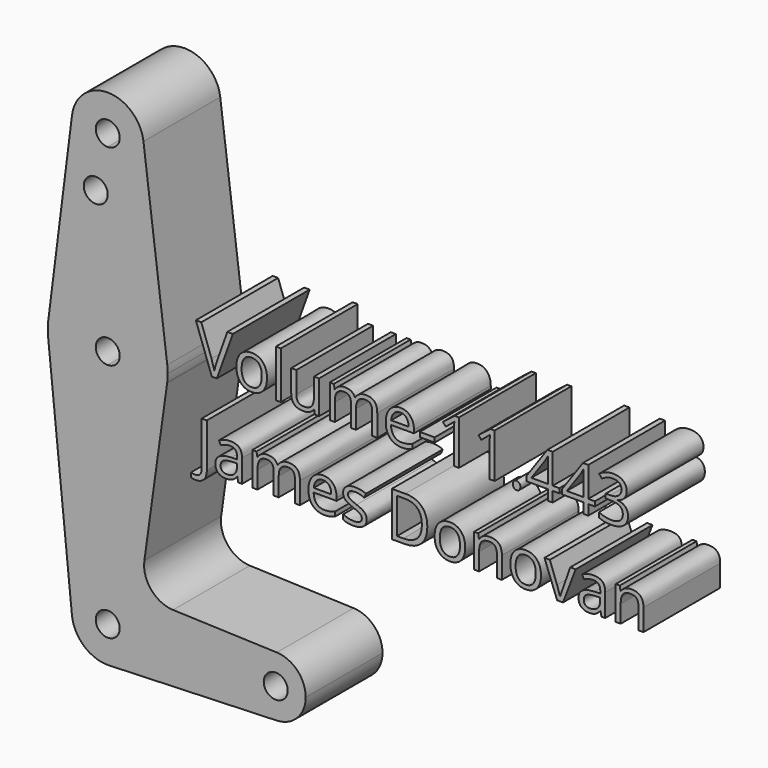
from build123d import *

# Parameters (mm, degrees)
F1_TEXT_SIZE = 16.465700335
F0_R         = 3.175
F2_DEPTH     = 25.4


# Not quite as in the source:
# - Text() gives the source's letters only with a copy of the font that has no kerning and outlines rounded to 1/6400 em; it was checked with that copy


with BuildPart() as f2:
    # F1 (on Front) + F0 (on Front) → F2 (new body)
    with BuildSketch(Plane.XZ):
        with Locations((-21.1360552348, 51.8487617373)):
            Text('Volume-11.443', F1_TEXT_SIZE, font='Open Sans', text_align=(TextAlign.LEFT, TextAlign.BOTTOM))
        with Locations((-21.1360552348, 29.4554092818)):
            Text('James Donovan', F1_TEXT_SIZE, font='Open Sans', text_align=(TextAlign.LEFT, TextAlign.BOTTOM))
    with BuildSketch(Plane.XZ):
        with BuildLine():
            ThreePointArc((-53.9002929642, 100.7426784498), (-51.59375, 93.2518581403), (-44.45, 90.0270534498))
            ThreePointArc((-44.45, 90.0270534498), (-37.7148079092, 92.816861359), (-34.925, 99.5520534498))
            ThreePointArc((-34.925, 99.5520534498), (-34.9436951058, 100.1485366917), (-34.9997070358, 100.7426784498))
            ThreePointArc((-34.9997070358, 100.7426784498), (-44.45, 109.0770534498), (-53.9002929642, 100.7426784498))
        make_face()
        with BuildLine():
            ThreePointArc((-41.275, 99.5520534498), (-42.2049359697, 97.3069894195), (-44.45, 96.3770534498))
            ThreePointArc((-44.45, 96.3770534498), (-46.6950640303, 101.79711748), (-41.275, 99.5520534498))
        make_face(mode=Mode.SUBTRACT)
        with BuildLine():
            ThreePointArc((-34.925, 99.5520534498), (-37.7148079092, 92.816861359), (-44.45, 90.0270534498))
            Line((-44.45, 90.0270534498), (-44.45, 85.2772534498))
            Line((-44.45, 85.2772534498), (-44.45, 64.6270534498))
            ThreePointArc((-44.45, 64.6270534498), (-33.9496744842, 60.6583034498), (-28.6995117263, 50.7364284498))
            Line((-28.6995117263, 50.7364284498), (-34.9997070358, 100.7426784498))
            ThreePointArc((-34.9997070358, 100.7426784498), (-34.9436951058, 100.1485366917), (-34.925, 99.5520534498))
        make_face()
        with BuildLine():
            Line((-44.45, 85.2772534498), (-44.45, 90.0270534498))
            ThreePointArc((-44.45, 90.0270534498), (-51.59375, 93.2518581403), (-53.9002929642, 100.7426784498))
            Line((-53.9002929642, 100.7426784498), (-60.2004882737, 50.7364284498))
            ThreePointArc((-60.2004882737, 50.7364284498), (-54.9503255158, 60.6583034498), (-44.45, 64.6270534498))
            Line((-44.45, 64.6270534498), (-44.45, 85.2772534498))
        make_face()
        with Locations((-47.625, 85.2772534498)):
            Circle(F0_R, mode=Mode.SUBTRACT)
        with BuildLine():
            ThreePointArc((-28.6995117263, 50.7364284498), (-33.9496744842, 60.6583034498), (-44.45, 64.6270534498))
            Line((-44.45, 64.6270534498), (-44.45, 51.9270534498))
            ThreePointArc((-44.45, 51.9270534498), (-42.2049359697, 50.99711748), (-41.275, 48.7520534498))
            ThreePointArc((-41.275, 48.7520534498), (-42.2049359697, 46.5069894195), (-44.45, 45.5770534498))
            Line((-44.45, 45.5770534498), (-44.45, 32.8770534498))
            ThreePointArc((-44.45, 32.8770534498), (-34.0672414406, 36.7431421879), (-28.7415746527, 46.4583668738))
            Line((-28.7415746527, 46.4583668738), (-28.7115456591, 46.6743913121))
            ThreePointArc((-28.7115456591, 46.6743913121), (-28.6091731961, 47.710981325), (-28.575, 48.7520534498))
            ThreePointArc((-28.575, 48.7520534498), (-28.6061585096, 49.7461921864), (-28.6995117263, 50.7364284498))
        make_face()
        with BuildLine():
            Line((-44.45, 51.9270534498), (-44.45, 64.6270534498))
            ThreePointArc((-44.45, 64.6270534498), (-54.9503255158, 60.6583034498), (-60.2004882737, 50.7364284498))
            ThreePointArc((-60.2004882737, 50.7364284498), (-60.3237438155, 48.9517589365), (-60.2454255641, 47.1645534498))
            ThreePointArc((-60.2454255641, 47.1645534498), (-55.0992737428, 36.9788383515), (-44.45, 32.8770534498))
            Line((-44.45, 32.8770534498), (-44.45, 45.5770534498))
            ThreePointArc((-44.45, 45.5770534498), (-47.625, 48.7520534498), (-44.45, 51.9270534498))
        make_face()
        with BuildLine():
            ThreePointArc((-44.45, 32.8770534498), (-55.0992737428, 36.9788383515), (-60.2454255641, 47.1645534498))
            Line((-60.2454255641, 47.1645534498), (-53.9272553384, -15.7004465502))
            ThreePointArc((-53.9272553384, -15.7004465502), (-51.513929059, -8.3583823045), (-44.45, -5.2229465502))
            Line((-44.45, -5.2229465502), (-44.45, 32.8770534498))
        make_face()
        with BuildLine():
            ThreePointArc((-28.7415746527, 46.4583668738), (-34.0672414406, 36.7431421879), (-44.45, 32.8770534498))
            Line((-44.45, 32.8770534498), (-44.45, -5.2229465502))
            ThreePointArc((-44.45, -5.2229465502), (-37.7148079092, -8.0127544594), (-34.925, -14.7479465502))
            Line((-34.925, -14.7479465502), (-7.9375, -14.7479465502))
            ThreePointArc((-7.9375, -14.7479465502), (-5.5115227815, -9.0359396455), (0.2834821429, -6.8155103466))
            Line((0.2834821429, -6.8155103466), (-27.1635488423, -5.8346334812))
            ThreePointArc((-27.1635488423, -5.8346334812), (-32.9680594139, -3.0018924799), (-34.7540975941, 3.2051061648))
            Line((-34.7540975941, 3.2051061648), (-28.7415746527, 46.4583668738))
        make_face()
        with BuildLine():
            ThreePointArc((-44.45, -5.2229465502), (-51.513929059, -8.3583823045), (-53.9272553384, -15.7004465502))
            ThreePointArc((-53.9272553384, -15.7004465502), (-50.7123833816, -21.9248664593), (-44.1098214286, -24.2668699946))
            ThreePointArc((-44.1098214286, -24.2668699946), (-37.5955917143, -21.361773888), (-34.925, -14.7479465502))
            Line((-34.925, -14.7479465502), (-41.275, -14.7479465502))
            ThreePointArc((-41.275, -14.7479465502), (-46.6950640303, -16.9930105805), (-44.45, -11.5729465502))
            Line((-44.45, -11.5729465502), (-44.45, -5.2229465502))
        make_face()
        with BuildLine():
            ThreePointArc((-28.7415746527, 46.4583668738), (-28.7261891651, 46.5663275225), (-28.7115456591, 46.6743913121))
            Line((-28.7115456591, 46.6743913121), (-28.7415746527, 46.4583668738))
        make_face()
        with BuildLine():
            ThreePointArc((-34.925, -14.7479465502), (-37.5955917143, -21.361773888), (-44.1098214286, -24.2668699946))
            Line((-44.1098214286, -24.2668699946), (0.2834821429, -22.6803827539))
            ThreePointArc((0.2834821429, -22.6803827539), (-5.5115227815, -20.4599534549), (-7.9375, -14.7479465502))
            Line((-7.9375, -14.7479465502), (-34.925, -14.7479465502))
        make_face()
        with BuildLine():
            ThreePointArc((-7.9375, -14.7479465502), (-5.5115227815, -20.4599534549), (0.2834821429, -22.6803827539))
            ThreePointArc((0.2834821429, -22.6803827539), (5.7120069047, -20.2594693317), (7.9375, -14.7479465502))
            ThreePointArc((7.9375, -14.7479465502), (5.7120069047, -9.2364237688), (0.2834821429, -6.8155103466))
            ThreePointArc((0.2834821429, -6.8155103466), (-5.5115227815, -9.0359396455), (-7.9375, -14.7479465502))
        make_face()
        with BuildLine():
            ThreePointArc((3.175, -14.7479465502), (0, -17.9229465502), (-3.175, -14.7479465502))
            ThreePointArc((-3.175, -14.7479465502), (0, -11.5729465502), (3.175, -14.7479465502))
        make_face(mode=Mode.SUBTRACT)
        with BuildLine():
            ThreePointArc((-34.925, -14.7479465502), (-37.7148079092, -8.0127544594), (-44.45, -5.2229465502))
            Line((-44.45, -5.2229465502), (-44.45, -11.5729465502))
            ThreePointArc((-44.45, -11.5729465502), (-42.2049359697, -12.50288252), (-41.275, -14.7479465502))
            Line((-41.275, -14.7479465502), (-34.925, -14.7479465502))
        make_face()
    extrude(amount=F2_DEPTH)


solid = f2.part
